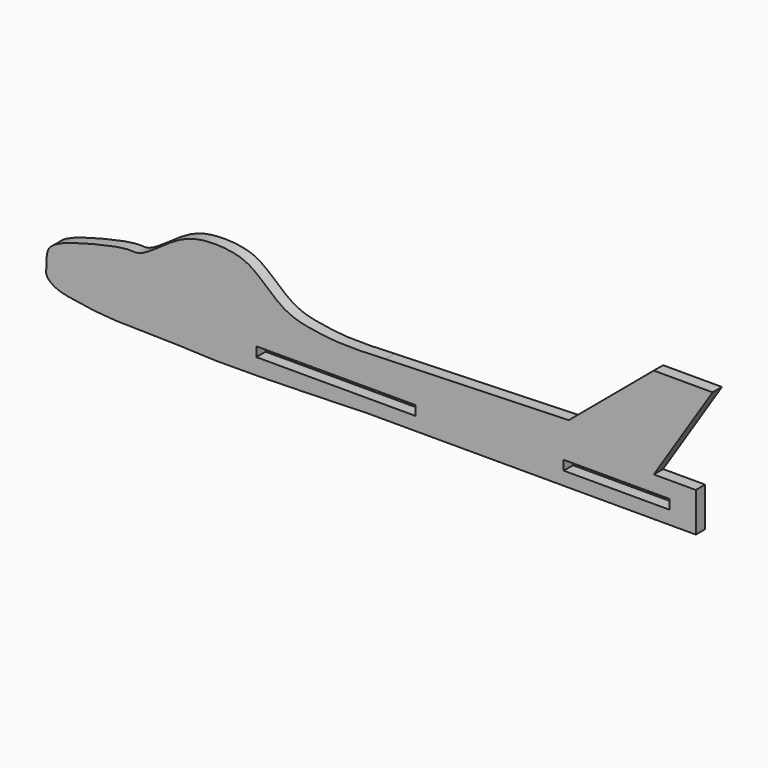
from build123d import *

# Parameters (mm, degrees)
F0_W     = 76.2
F0_H     = 4.572
F0_W_2   = 50.8
F1_DEPTH = 5.588


with BuildPart() as f1:
    # F0 (on Front) → F1 (new body)
    with BuildSketch(Plane.XZ):
        with BuildLine():
            add(Edge.make_bspline(
                [(5.1831402816, 34.1174341738), (5.3384693548, 35.6871684741), (5.6891144403, 39.2307395946), (13.0501725287, 43.2881274426), (25.0316226376, 46.7321573297), (44.2363434166, 51.2689101035), (50.3802908007, 49.1951338229), (64.9303946793, 60.9512807395), (75.0422661497, 65.3864074535), (85.1028309036, 66.5640317959), (96.9584527395, 65.5237584095), (105.8803939506, 61.147117083), (118.6971984759, 48.0707941944), (131.9122664086, 45.3132218555), (146.7798154171, 43.322102422), (160.2514465699, 43.9344012555), (167.594820261, 44.2681647837)],
                knots=[0, 0, 0, 0, 0.0440043821, 0.0993369754, 0.1747943401, 0.2640154465, 0.3145440637, 0.3997217371, 0.4694587784, 0.5335500622, 0.6027058317, 0.6673380282, 0.7532073344, 0.8275843868, 0.9060164086, 1, 1, 1, 1], degree=3))
            add(Edge.make_bspline(
                [(5.1831402816, 34.1174341738), (5.2429216667, 33.0711454398), (5.3692739062, 30.859739255), (4.2589819802, 26.3812506128), (9.9094275754, 22.104272954), (18.5984539101, 20.5857647973), (31.010439708, 18.6841603181), (46.1342712862, 18.0647561335), (65.9300368986, 18.1659522123), (82.3554701732, 16.797902378), (120.284901018, 17.3621123501), (144.9557022783, 18.1519831985), (157.389998436, 18.5500849038)],
                knots=[0, 0, 0, 0, 0.0481445289, 0.1017569105, 0.1674244019, 0.2470873084, 0.3410679714, 0.446256147, 0.563098919, 0.6723348225, 0.8348539306, 1, 1, 1, 1], degree=3))
            Line((157.389998436, 18.5500849038), (316.2764310837, 18.5500849038))
            Line((316.2764310837, 18.5500849038), (316.2764310837, 37.3842418194))
            Line((316.2764310837, 37.3842418194), (296.1356043816, 37.3842418194))
            Line((296.1356043816, 37.3842418194), (324.3215382099, 81.1939239502))
            Line((324.3215382099, 81.1939239502), (296.1356043816, 81.1939239502))
            Line((296.1356043816, 81.1939239502), (255.4179131985, 47.0325164497))
            Line((255.4179131985, 47.0325164497), (167.594820261, 44.2681647837))
        make_face()
        with Locations((143.7541278958, 27.2327175454)):
            Rectangle(F0_W, F0_H, mode=Mode.SUBTRACT)
        with Locations((278.3746890068, 27.2327175454)):
            Rectangle(F0_W_2, F0_H, mode=Mode.SUBTRACT)
    extrude(amount=F1_DEPTH)


solid = f1.part
